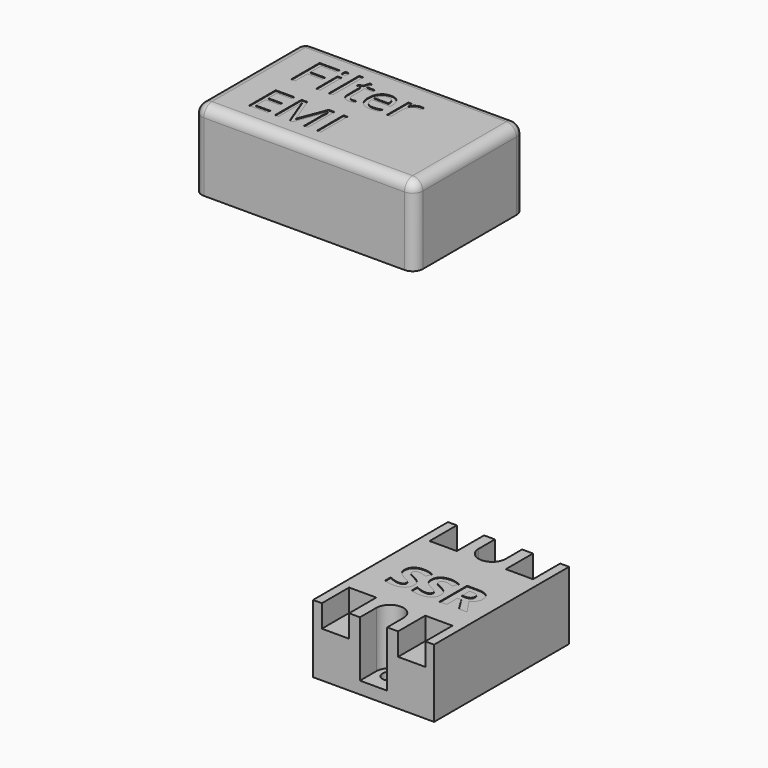
from build123d import *

# Parameters (mm, degrees)
F1_DEPTH        = 25.4
F0_R            = 2.8000025437
F0_R_2          = 2.5146
F2_DEPTH        = 4.572
F3_W            = 10.16
F3_H            = 12.7
F4_DEPTH        = 8.382
F3_TEXT_SIZE    = 18.0945576479
F5_DEPTH        = 0.254
F7_W            = 82.55
F7_H            = 51.308
F8_DEPTH        = 29.464
F9_R            = 3.81
F10_TEXT_SIZE   = 18.6243016894
F10_TEXT_SIZE_2 = 17.3826821588
F11_DEPTH       = 0.254


# Not quite as in the source:
# - Text() gives the source's letters only with a copy of the font that has no kerning and outlines rounded to 1/6400 em; it was checked with that copy


with BuildPart() as f1:
    # F0 (on Top) → F1 (new body)
    with BuildSketch(Plane.XY):
        with BuildLine():
            Line((0, 62.992), (0, 0))
            Line((0, 0), (17.526, 0))
            Line((17.526, 0), (17.526, 7.62))
            ThreePointArc((17.526, 7.62), (22.606, 12.7), (27.686, 7.62))
            Line((27.686, 7.62), (27.686, 0))
            Line((27.686, 0), (45.212, 0))
            Line((45.212, 0), (45.212, 62.992))
            Line((45.212, 62.992), (27.686, 62.992))
            Line((27.686, 62.992), (27.686, 55.372))
            ThreePointArc((27.686, 55.372), (22.606, 50.292), (17.526, 55.372))
            Line((17.526, 55.372), (17.526, 62.992))
            Line((17.526, 62.992), (0, 62.992))
        make_face()
    extrude(amount=F1_DEPTH)

    # F0 (on Top) → F2 (join)
    with BuildSketch(Plane.XY):
        with BuildLine():
            Line((17.526, 7.62), (17.526, 0))
            Line((17.526, 0), (27.686, 0))
            Line((27.686, 0), (27.686, 7.62))
            ThreePointArc((27.686, 7.62), (22.606, 12.7), (17.526, 7.62))
        make_face()
        with Locations((22.606, 7.62)):
            Circle(F0_R, mode=Mode.SUBTRACT)
        with BuildLine():
            Line((27.686, 62.992), (17.526, 62.992))
            Line((17.526, 62.992), (17.526, 55.372))
            ThreePointArc((17.526, 55.372), (22.606, 50.292), (27.686, 55.372))
            Line((27.686, 55.372), (27.686, 62.992))
        make_face()
        with Locations((22.606, 55.372)):
            Circle(F0_R_2, mode=Mode.SUBTRACT)
    extrude(amount=F2_DEPTH)

    # F3 (on face) → F4 (cut)
    with BuildSketch(Plane.XY.offset(25.4)):
        with Locations((36.83, 6.35)):
            Rectangle(F3_W, F3_H)
        with Locations((8.382, 6.35)):
            Rectangle(F3_W, F3_H)
        with Locations((8.382, 56.642)):
            Rectangle(F3_W, F3_H)
        with Locations((36.83, 56.642)):
            Rectangle(F3_W, F3_H)
    extrude(amount=-F4_DEPTH, mode=Mode.SUBTRACT)

    # F3 (on face) → F5 (cut)
    with BuildSketch(Plane.XY.offset(25.4)):
        with Locations((7.92457629, 22.1451260149)):
            Text('SSR', F3_TEXT_SIZE, font='Open Sans', font_style=FontStyle.BOLD, text_align=(TextAlign.LEFT, TextAlign.BOTTOM))
    extrude(amount=-F5_DEPTH, mode=Mode.SUBTRACT)


with BuildPart() as f8:
    # F7 (on offset) → F8 (new body)
    with BuildSketch(Plane.XY.offset(152.4)):
        with Locations((5.5890811741, 14.5285145872)):
            Rectangle(F7_W, F7_H)
    extrude(amount=F8_DEPTH)

    # F9
    f9_edges = [f8.edges().sort_by_distance(p)[0] for p in [
        (5.589081, -11.125485, 181.864),
        (46.864081, 14.528515, 181.864),
        (5.589081, 40.182515, 181.864),
        (46.864081, 40.182515, 167.132),
        (-35.685919, 40.182515, 167.132),
        (46.864081, -11.125485, 167.132),
        (-35.685919, 14.528515, 181.864),
        (-35.685919, -11.125485, 167.132),
    ]]
    fillet(f9_edges, radius=F9_R)

    # F10 (on face) → F11 (cut)
    with BuildSketch(Plane.XY.offset(181.864)):
        with Locations((-24.4350843132, 18.0283244699)):
            Text('Filter', F10_TEXT_SIZE, font='Open Sans', text_align=(TextAlign.LEFT, TextAlign.BOTTOM))
        with Locations((-23.541117087, -2.5329052005)):
            Text('EMI', F10_TEXT_SIZE_2, font='Open Sans', text_align=(TextAlign.LEFT, TextAlign.BOTTOM))
    extrude(amount=-F11_DEPTH, mode=Mode.SUBTRACT)


solid = Compound([f1.part, f8.part])
